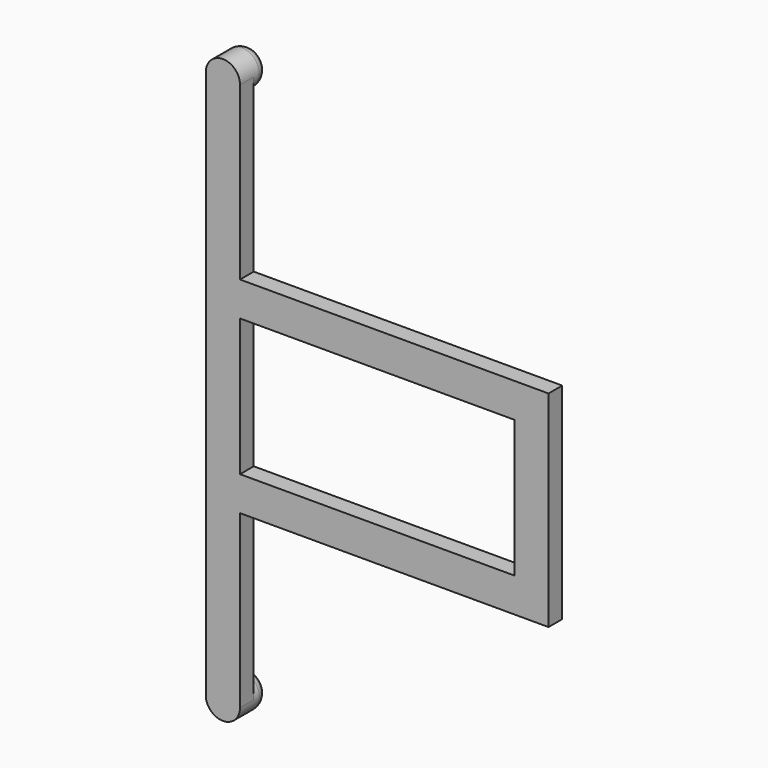
from build123d import *

# Parameters (mm, degrees)
F0_DEPTH = 3.175
F1_R     = 3.175
F4_DEPTH = 6.35
F2_R     = 1.905


# Not quite as in the source:
# - a length typed as a fraction of an inch, garbled in the dataset ("3 / 203.2 mm" for 3/8 in), is restored


with BuildPart() as f0:
    # F3 (on Front) → F0 (new body)
    with BuildSketch(Plane.XZ):
        Polygon((6.35, 50.8), (0, 50.8), (0, 0), (0, -50.8), (6.35, -50.8), (6.35, -19.05), (63.5, -19.05), (63.5, 19.05), (6.35, 19.05), align=None)
        Polygon((6.35, -12.7), (6.35, 0), (6.35, 12.7), (57.15, 12.7), (57.15, -12.7), align=None, mode=Mode.SUBTRACT)
    extrude(amount=F0_DEPTH)

    # F1 (on face) → F4 (join)
    with BuildSketch(Plane.XZ.offset(3.175)):
        with Locations((3.175, -50.8)):
            Circle(F1_R)
        with Locations((3.175, 50.8)):
            Circle(F1_R)
    extrude(amount=-F4_DEPTH)

    # F2
    f2_edges = [f0.edges().sort_by_distance(p)[0] for p in [
        (0, 3.175, 50.8),
        (0, 3.175, -50.8),
    ]]
    fillet(f2_edges, radius=F2_R)


solid = f0.part
